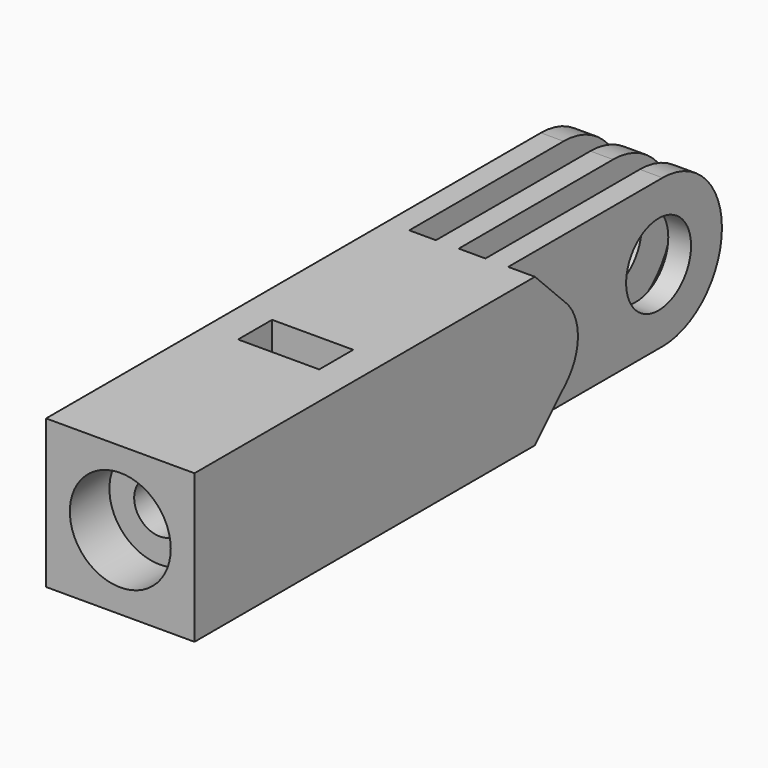
from build123d import *

# Parameters (mm, degrees)
F1_DEPTH       = 15
F3_D           = 5.2
F3_DEPTH       = 30
F3_CBORE_D     = 10.2
F3_CBORE_DEPTH = 5
F3_TIP         = 1.5622376095
F4_W           = 8.2
F4_H           = 4.3
F5_DEPTH       = 12.4
F6_R           = 4.1
F7_DEPTH       = 25
F8_R           = 7.5
F9_R           = 7.5
F10_R          = 7.49999
F11_SIZE       = 11
F12_T1_DEPTH   = 2.7
F12_T3_DEPTH   = 2.7
F12_T5_DEPTH   = 30.9885128676
F12_T10_DEPTH  = 59.2770257353
F12_T15_DEPTH  = 59.2770257353
F12_T21_DEPTH  = 59.2770257353
F12_T26_DEPTH  = 59.2770257353
F12_T32_DEPTH  = 59.2770257353
F12_T38_DEPTH  = 59.2770257353
F13_R          = 5


# Not quite as in the source:
# - a fillet or chamfer that OpenCascade refuses, or shapes differently, is made with other operations: its cross-section is extruded or revolved along the edge and cut away or added
# - a fillet or chamfer is up to 0.001 mm smaller than in the source, because OpenCascade refuses the exact size


with BuildPart() as f1:
    # F0 (on Top) → F1 (new body)
    with BuildSketch(Plane.XY):
        Polygon((-7.0407824647, 62.3018580846), (-7.0407824647, -7.6981419154), (7.9592175353, -7.6981419154), (7.9592175353, 46.3018580846), (5.2592175353, 46.3018580846), (5.2592175353, 62.3018580846), (2.9592175353, 62.3018580846), (2.9592175353, 46.3018580846), (0.2592175353, 46.3018580846), (0.2592175353, 62.3018580846), (-2.0407824647, 62.3018580846), (-2.0407824647, 46.3018580846), (-4.7407824647, 46.3018580846), (-4.7407824647, 62.3018580846), align=None)
    extrude(amount=F1_DEPTH)

    # F3
    with Locations(Plane.XZ.offset(7.6981419154)):
        with Locations((0.4592175353, 7.5)):
            CounterBoreHole(F3_D / 2, F3_CBORE_D / 2, F3_CBORE_DEPTH, depth=F3_DEPTH)
            with Locations((0, 0, -(F3_DEPTH + F3_TIP / 2))):  # 118° drill point
                Cone(0, F3_D / 2, F3_TIP, mode=Mode.SUBTRACT)

    # F4 (on face) → F5 (cut)
    with BuildSketch(Plane.XY.offset(15)):
        with Locations((0.4592175353, 14.4518580846)):
            Rectangle(F4_W, F4_H)
    extrude(amount=-F5_DEPTH, mode=Mode.SUBTRACT)

    # F6 (on face) → F7 (cut)
    with BuildSketch(Plane.YZ.offset(5.2592175353)):
        with Locations((54.3018580846, 7.5)):
            Circle(F6_R)
    extrude(amount=-F7_DEPTH, mode=Mode.SUBTRACT)

    # F8
    f8_edges = [f1.edges().sort_by_distance(p)[0] for p in [
        (-5.890782, 62.301858, 0),
    ]]
    fillet(f8_edges, radius=F8_R)

    # F9
    f9_edges = [f1.edges().sort_by_distance(p)[0] for p in [
        (-0.890782, 62.301858, 0),
        (4.109218, 62.301858, 0),
    ]]
    fillet(f9_edges, radius=F9_R)

    # F10 (radius 7.5 in the source; OpenCascade refuses exactly that, so slightly less here)
    f10_edges = [f1.edges().sort_by_distance(p)[0] for p in [
        (-5.890782, 62.301858, 15),
        (-0.890782, 62.301858, 15),
        (4.109218, 62.301858, 15),
    ]]
    fillet(f10_edges, radius=F10_R)

    # F11
    f11_edges = [f1.edges().sort_by_distance(p)[0] for p in [
        (-3.390782, 46.301858, 15),
        (1.609218, 46.301858, 15),
        (6.609218, 46.301858, 15),
    ]]
    chamfer(f11_edges, length=F11_SIZE)

    # F12: chamfer of 11 on 3 edges, made by hand

    # F12_s2 → F12_t1 (cut)
    with BuildSketch(Plane.YZ.offset(-4.7407824647)):
        Polygon((46.3018580846, 11), (35.3018580846, 0), (46.3018580846, 0), align=None)
    extrude(amount=F12_T1_DEPTH, mode=Mode.SUBTRACT)

    # F12_s4 → F12_t3 (cut)
    with BuildSketch(Plane.YZ.offset(0.2592175353)):
        Polygon((35.3018580846, 0), (46.3018580846, 11), (46.3018580846, 0), align=None)
    extrude(amount=F12_T3_DEPTH, mode=Mode.SUBTRACT)

    # F12_s6 → F12_t5 (cut)
    with BuildSketch(Plane.YZ.offset(5.2592175353)):
        Polygon((35.3018580846, 0), (46.3018580846, 11), (46.3018580846, 0), align=None)
    extrude(amount=F12_T5_DEPTH, mode=Mode.SUBTRACT)


with BuildPart() as f12_tool8:
    # F12_s9 → F12_t10 (new body)
    with BuildSketch(Plane.YZ.offset(26.247730403)):
        Polygon((46.3018580846, 11), (35.3018580846, 0), (46.3018580846, 0), align=None)
    extrude(amount=-F12_T10_DEPTH)

    split(bisect_by=Plane.YZ.offset(5.2592175353), keep=Keep.TOP)


with BuildPart() as f1_1:
    add(f1.part)

    # F12_t7: cut F12_tool8
    add(f12_tool8.part, mode=Mode.SUBTRACT)


with BuildPart() as f12_tool13:
    # F12_s14 → F12_t15 (new body)
    with BuildSketch(Plane.YZ.offset(26.247730403)):
        Polygon((46.3018580846, 11), (35.3018580846, 0), (46.3018580846, 0), align=None)
    extrude(amount=-F12_T15_DEPTH)

    split(bisect_by=Plane.YZ.offset(0.2592175353), keep=Keep.TOP)

    split(bisect_by=Plane.YZ.offset(2.9592175353), keep=Keep.BOTTOM)


with BuildPart() as f1_2:
    add(f1_1.part)

    # F12_t12: cut F12_tool13
    add(f12_tool13.part, mode=Mode.SUBTRACT)


with BuildPart() as f12_tool19:
    # F12_s20 → F12_t21 (new body)
    with BuildSketch(Plane.YZ.offset(31.247730403)):
        Polygon((35.3018580846, 0), (46.3018580846, 11), (46.3018580846, 0), align=None)
    extrude(amount=-F12_T21_DEPTH)

    split(bisect_by=Plane.YZ.offset(5.2592175353), keep=Keep.TOP)


with BuildPart() as f1_3:
    add(f1_2.part)

    # F12_t18: cut F12_tool19
    add(f12_tool19.part, mode=Mode.SUBTRACT)


with BuildPart() as f12_tool24:
    # F12_s25 → F12_t26 (new body)
    with BuildSketch(Plane.YZ.offset(31.247730403)):
        Polygon((35.3018580846, 0), (46.3018580846, 11), (46.3018580846, 0), align=None)
    extrude(amount=-F12_T26_DEPTH)

    split(bisect_by=Plane.YZ.offset(-2.0407824647), keep=Keep.BOTTOM)

    split(bisect_by=Plane.YZ.offset(-4.7407824647), keep=Keep.TOP)


with BuildPart() as f1_4:
    add(f1_3.part)

    # F12_t23: cut F12_tool24
    add(f12_tool24.part, mode=Mode.SUBTRACT)


with BuildPart() as f12_tool30:
    # F12_s31 → F12_t32 (new body)
    with BuildSketch(Plane.YZ.offset(36.247730403)):
        Polygon((35.3018580846, 0), (46.3018580846, 11), (46.3018580846, 0), align=None)
    extrude(amount=-F12_T32_DEPTH)

    split(bisect_by=Plane.YZ.offset(0.2592175353), keep=Keep.TOP)

    split(bisect_by=Plane.YZ.offset(2.9592175353), keep=Keep.BOTTOM)


with BuildPart() as f1_5:
    add(f1_4.part)

    # F12_t29: cut F12_tool30
    add(f12_tool30.part, mode=Mode.SUBTRACT)


with BuildPart() as f12_tool36:
    # F12_s37 → F12_t38 (new body)
    with BuildSketch(Plane.YZ.offset(36.247730403)):
        Polygon((35.3018580846, 0), (46.3018580846, 11), (46.3018580846, 0), align=None)
    extrude(amount=-F12_T38_DEPTH)

    split(bisect_by=Plane.YZ.offset(-2.0407824647), keep=Keep.BOTTOM)

    split(bisect_by=Plane.YZ.offset(-4.7407824647), keep=Keep.TOP)


with BuildPart() as f1_6:
    add(f1_5.part)

    # F12_t35: cut F12_tool36
    add(f12_tool36.part, mode=Mode.SUBTRACT)

    # F13
    f13_edges = [f1_6.edges().sort_by_distance(p)[0] for p in [
        (1.609218, 42.801858, 7.5),
        (6.609218, 42.801858, 7.5),
        (-3.390782, 42.801858, 7.5),
    ]]
    fillet(f13_edges, radius=F13_R)


solid = f1_6.part
